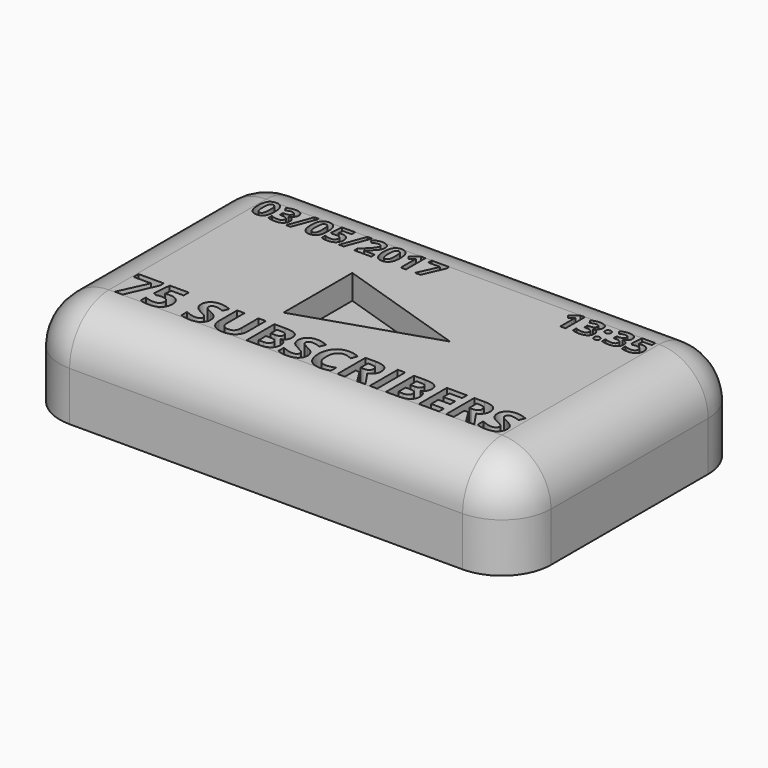
from build123d import *

# Parameters (mm, degrees)
F0_W           = 100
F0_H           = 60
F1_DEPTH       = 20
F2_R           = 10
F5_TEXT_SIZE   = 9.9659367397
F5_TEXT_SIZE_2 = 6.9444444444
F6_DEPTH       = 5


# Not quite as in the source:
# - Text() gives the source's letters only with a copy of the font that has no kerning and outlines rounded to 1/6400 em; it was checked with that copy


with BuildPart() as f1:
    # F0 (on Top) → F1 (new body)
    with BuildSketch(Plane.XY):
        Rectangle(F0_W, F0_H)
    extrude(amount=F1_DEPTH)

    # F2
    f2_edges = [f1.edges().sort_by_distance(p)[0] for p in [
        (50, 0, 20),
        (0, 30, 20),
        (-50, 0, 20),
        (0, -30, 20),
        (50, -30, 10),
        (-50, -30, 10),
        (-50, 30, 10),
        (50, 30, 10),
    ]]
    fillet(f2_edges, radius=F2_R)

    # F4 (on face) + F5 (on face) → F6 (cut)
    with BuildSketch(Plane.XY.offset(20)):
        Polygon((13.4529350325, 0), (-13.4529350325, 8.7530948222), (-13.4529350325, -8.7530948222), align=None)
    with BuildSketch(Plane.XY.offset(20)):
        with Locations((-39.9853882598, -19.8844364394)):
            Text('75 SUBSCRIBERS', F5_TEXT_SIZE, font='Open Sans', font_style=FontStyle.BOLD, text_align=(TextAlign.LEFT, TextAlign.BOTTOM))
        with Locations((-39.9300865829, 15.0066305697)):
            Text('03/05/2017', F5_TEXT_SIZE_2, font='Open Sans', font_style=FontStyle.BOLD, text_align=(TextAlign.LEFT, TextAlign.BOTTOM))
        with Locations((22.0607658972, 15.0066296384)):
            Text('13:35', F5_TEXT_SIZE_2, font='Open Sans', font_style=FontStyle.BOLD, text_align=(TextAlign.LEFT, TextAlign.BOTTOM))
    extrude(amount=-F6_DEPTH, mode=Mode.SUBTRACT)


solid = f1.part
